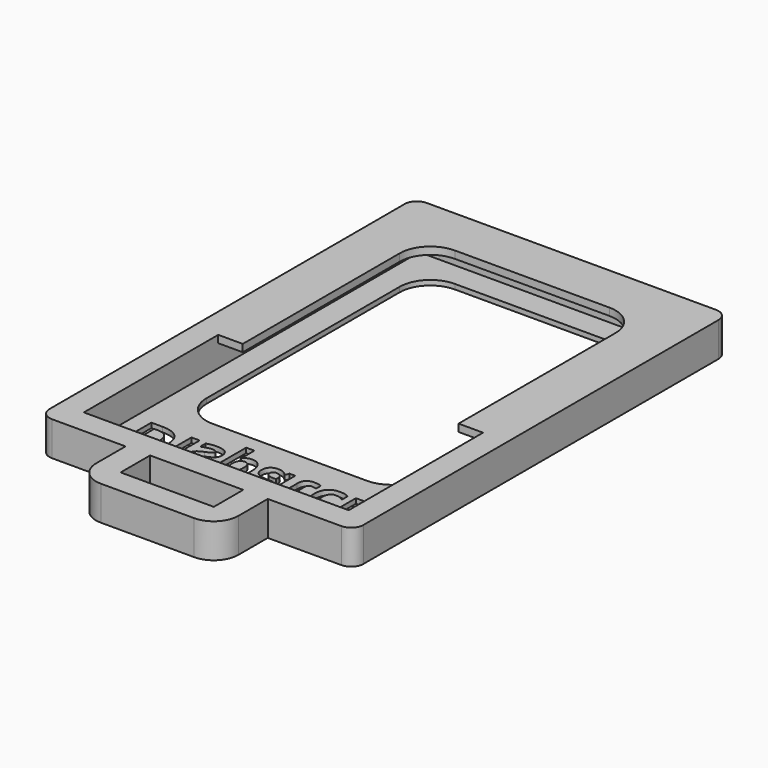
from build123d import *

# Parameters (mm, degrees)
F0_W         = 65.024
F0_H         = 97.028
F0_W_2       = 54.864
F0_H_2       = 86.868
F1_DEPTH     = 7.112
F2_W         = 54.864
F2_H         = 86.868
F3_DEPTH     = 1.016
F4_TEXT_SIZE = 11.4035482208
F5_DEPTH     = 25.4
F7_DEPTH     = 7.112
F9_DEPTH     = 1.524
F10_R        = 2.54


# Not quite as in the source:
# - Text() gives the source's letters only with a copy of the font that has no kerning and outlines rounded to 1/6400 em; it was checked with that copy


with BuildPart() as f1:
    # F0 (on Top) → F1 (new body)
    with BuildSketch(Plane.XY):
        with Locations((-27.432, -43.434)):
            Rectangle(F0_W, F0_H)
        with Locations((-27.432, -43.434)):
            Rectangle(F0_W_2, F0_H_2, mode=Mode.SUBTRACT)
    extrude(amount=F1_DEPTH)

    # F6 (on face) → F7 (join, through all)
    with BuildSketch(Plane.XY.offset(7.112)):
        with BuildLine():
            Line((-37.084, -91.948), (-42.164, -91.948))
            Line((-42.164, -91.948), (-42.164, -99.568))
            ThreePointArc((-42.164, -99.568), (-40.6761024484, -103.1601024484), (-37.084, -104.648))
            Line((-37.084, -104.648), (-17.78, -104.648))
            ThreePointArc((-17.78, -104.648), (-14.1878975516, -103.1601024484), (-12.7, -99.568))
            Line((-12.7, -99.568), (-12.7, -91.948))
            Line((-12.7, -91.948), (-17.78, -91.948))
            Line((-17.78, -91.948), (-17.78, -99.568))
            Line((-17.78, -99.568), (-37.084, -99.568))
            Line((-37.084, -99.568), (-37.084, -91.948))
        make_face()
    extrude(amount=-F7_DEPTH)

    # F8 (on face) → F9 (join)
    with BuildSketch(Plane.XY.offset(7.112)):
        with BuildLine():
            Line((0, -52.07), (0, 0))
            Line((0, 0), (-54.864, 0))
            Line((-54.864, 0), (-54.864, -52.07))
            Line((-54.864, -52.07), (-49.784, -52.07))
            Line((-49.784, -52.07), (-49.784, -11.43))
            ThreePointArc((-49.784, -11.43), (-47.9241280605, -6.9398719395), (-43.434, -5.08))
            Line((-43.434, -5.08), (-11.43, -5.08))
            ThreePointArc((-11.43, -5.08), (-6.9398719395, -6.9398719395), (-5.08, -11.43))
            Line((-5.08, -11.43), (-5.08, -52.07))
            Line((-5.08, -52.07), (0, -52.07))
        make_face()
    extrude(amount=-F9_DEPTH)

    # F10
    f10_edges = [f1.edges().sort_by_distance(p)[0] for p in [
        (-59.944, -91.948, 3.556),
        (5.08, -91.948, 3.556),
        (-59.944, 5.08, 3.556),
        (5.08, 5.08, 3.556),
    ]]
    fillet(f10_edges, radius=F10_R)


with BuildPart() as f3:
    # F2 (on face) → F3 (new body)
    with BuildSketch(Plane(origin=(0, 0, 0), x_dir=(1, 0, 0), z_dir=(0, 0, -1))):
        with Locations((-27.432, 43.434)):
            Rectangle(F2_W, F2_H)
        with BuildLine():
            Line((-11.43, 5.08), (-43.434, 5.08))
            ThreePointArc((-43.434, 5.08), (-47.9241280605, 6.9398719395), (-49.784, 11.43))
            Line((-49.784, 11.43), (-49.784, 61.468))
            ThreePointArc((-49.784, 61.468), (-47.9241280605, 65.9581280605), (-43.434, 67.818))
            Line((-43.434, 67.818), (-11.43, 67.818))
            ThreePointArc((-11.43, 67.818), (-6.9398719395, 65.9581280605), (-5.08, 61.468))
            Line((-5.08, 61.468), (-5.08, 11.43))
            ThreePointArc((-5.08, 11.43), (-6.9398719395, 6.9398719395), (-11.43, 5.08))
        make_face(mode=Mode.SUBTRACT)
    extrude(amount=-F3_DEPTH)

    # F4 (on face) → F5 (cut)
    with BuildSketch(Plane(origin=(0, 0, 0), x_dir=(1, 0, 0), z_dir=(0, 0, -1))):
        with Locations((-52.4443164468, 73.6933797598)):
            Text('Dispatch', F4_TEXT_SIZE, font='Open Sans', font_style=FontStyle.BOLD, text_align=(TextAlign.LEFT, TextAlign.BOTTOM))
    extrude(amount=-F5_DEPTH, mode=Mode.SUBTRACT)


solid = Compound([f1.part, f3.part])
